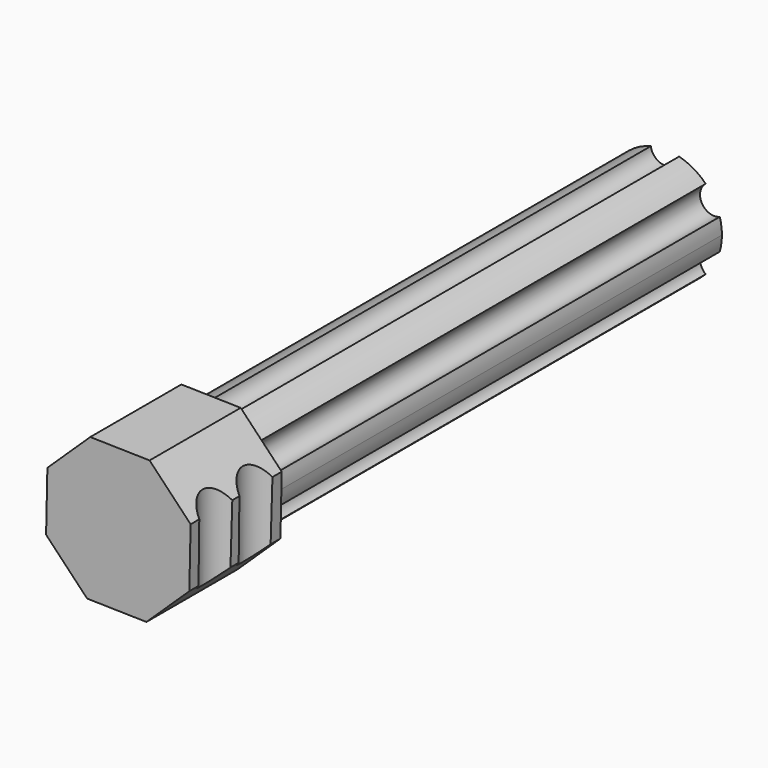
from build123d import *

# Parameters (mm, degrees)
F1_DEPTH        = 50.8
F3_DEPTH        = 10.16
F4_R            = 2.032
F5_DEPTH        = 12.7
F5_COPIES_COUNT = 2


# Not quite as in the source:
# - a pattern or mirror of a feature is missing from the dataset's text; its kind, count and spacing are read off the source's solid


with BuildPart() as f1:
    # F0 (on Front) → F1 (new body)
    with BuildSketch(Plane.XZ):
        with BuildLine():
            ThreePointArc((4.8919470493, -1.3693991626), (5.0327671817, -0.6911255275), (5.08, 0))
            ThreePointArc((5.08, 0), (5.0327671817, 0.6911255275), (4.8919470493, 1.3693991626))
            ThreePointArc((4.8919470493, 1.3693991626), (3.2995567884, 1.905), (3.6319079874, 3.5518508374))
            ThreePointArc((3.6319079874, 3.5518508374), (2.54, 4.3994090512), (1.2600390619, 4.92125))
            ThreePointArc((1.2600390619, 4.92125), (0, 3.81), (-1.2600390619, 4.92125))
            ThreePointArc((-1.2600390619, 4.92125), (-2.54, 4.3994090512), (-3.6319079874, 3.5518508374))
            ThreePointArc((-3.6319079874, 3.5518508374), (-3.2619499638, 3.1048777076), (-3.1294090512, 2.54))
            ThreePointArc((-3.1294090512, 2.54), (-3.6967794395, 1.4820720115), (-4.8919470493, 1.3693991626))
            ThreePointArc((-4.8919470493, 1.3693991626), (-5.08, 0), (-4.8919470493, -1.3693991626))
            ThreePointArc((-4.8919470493, -1.3693991626), (-3.6967794395, -1.4820720115), (-3.1294090512, -2.54))
            ThreePointArc((-3.1294090512, -2.54), (-3.2619499638, -3.1048777076), (-3.6319079874, -3.5518508374))
            ThreePointArc((-3.6319079874, -3.5518508374), (-2.54, -4.3994090512), (-1.2600390619, -4.92125))
            ThreePointArc((-1.2600390619, -4.92125), (0, -3.81), (1.2600390619, -4.92125))
            ThreePointArc((1.2600390619, -4.92125), (2.54, -4.3994090512), (3.6319079874, -3.5518508374))
            ThreePointArc((3.6319079874, -3.5518508374), (3.2995567884, -1.905), (4.8919470493, -1.3693991626))
        make_face()
    extrude(amount=F1_DEPTH)

    # F2 (on face) → F3 (join)
    with BuildSketch(Plane.XZ.offset(50.8)):
        Polygon((-2.506501507, 6.4478875138), (-6.331709198, 2.7869807727), (-6.4478875138, -2.506501507), (-2.7869807727, -6.331709198), (2.506501507, -6.4478875138), (6.331709198, -2.7869807727), (6.4478875138, 2.506501507), (2.7869807727, 6.331709198), align=None)
        with BuildLine():
            ThreePointArc((4.8919470493, 1.3693991626), (5.08, 0), (4.8919470493, -1.3693991626))
            ThreePointArc((4.8919470493, -1.3693991626), (3.2995567884, -1.905), (3.6319079874, -3.5518508374))
            ThreePointArc((3.6319079874, -3.5518508374), (2.54, -4.3994090512), (1.2600390619, -4.92125))
            ThreePointArc((1.2600390619, -4.92125), (0, -3.81), (-1.2600390619, -4.92125))
            ThreePointArc((-1.2600390619, -4.92125), (-2.54, -4.3994090512), (-3.6319079874, -3.5518508374))
            ThreePointArc((-3.6319079874, -3.5518508374), (-3.2995567884, -1.905), (-4.8919470493, -1.3693991626))
            ThreePointArc((-4.8919470493, -1.3693991626), (-5.08, 0), (-4.8919470493, 1.3693991626))
            ThreePointArc((-4.8919470493, 1.3693991626), (-3.2995567884, 1.905), (-3.6319079874, 3.5518508374))
            ThreePointArc((-3.6319079874, 3.5518508374), (-2.54, 4.3994090512), (-1.2600390619, 4.92125))
            ThreePointArc((-1.2600390619, 4.92125), (0, 3.81), (1.2600390619, 4.92125))
            ThreePointArc((1.2600390619, 4.92125), (2.54, 4.3994090512), (3.6319079874, 3.5518508374))
            ThreePointArc((3.6319079874, 3.5518508374), (3.2995567884, 1.905), (4.8919470493, 1.3693991626))
        make_face(mode=Mode.SUBTRACT)
        with BuildLine():
            ThreePointArc((3.6319079874, -3.5518508374), (3.2995567884, -1.905), (4.8919470493, -1.3693991626))
            ThreePointArc((4.8919470493, -1.3693991626), (5.08, 0), (4.8919470493, 1.3693991626))
            ThreePointArc((4.8919470493, 1.3693991626), (3.2995567884, 1.905), (3.6319079874, 3.5518508374))
            ThreePointArc((3.6319079874, 3.5518508374), (2.54, 4.3994090512), (1.2600390619, 4.92125))
            ThreePointArc((1.2600390619, 4.92125), (0, 3.81), (-1.2600390619, 4.92125))
            ThreePointArc((-1.2600390619, 4.92125), (-2.54, 4.3994090512), (-3.6319079874, 3.5518508374))
            ThreePointArc((-3.6319079874, 3.5518508374), (-3.2995567884, 1.905), (-4.8919470493, 1.3693991626))
            ThreePointArc((-4.8919470493, 1.3693991626), (-5.08, 0), (-4.8919470493, -1.3693991626))
            ThreePointArc((-4.8919470493, -1.3693991626), (-3.2995567884, -1.905), (-3.6319079874, -3.5518508374))
            ThreePointArc((-3.6319079874, -3.5518508374), (-2.54, -4.3994090512), (-1.2600390619, -4.92125))
            ThreePointArc((-1.2600390619, -4.92125), (0, -3.81), (1.2600390619, -4.92125))
            ThreePointArc((1.2600390619, -4.92125), (2.54, -4.3994090512), (3.6319079874, -3.5518508374))
        make_face()
    extrude(amount=F3_DEPTH)

    # F4 (on Top) → F5 (cut, symmetric)
    with BuildSketch(Plane.XY):
        with Locations((-7.3084752075, -53.6753074016)):
            Circle(F4_R)
        with Locations((-7.3084752075, -58.1539007338)):
            Circle(F4_R)
    f5 = extrude(amount=F5_DEPTH, both=True, mode=Mode.SUBTRACT)

    # F5_copies: F5 ×2 about axis
    f5_copies_axis = Axis((0, 0, 0), (0, 1, 0))
    for i in range(1, F5_COPIES_COUNT):
        add(f5.rotate(f5_copies_axis, i * 360 / F5_COPIES_COUNT), mode=Mode.SUBTRACT)


solid = f1.part
